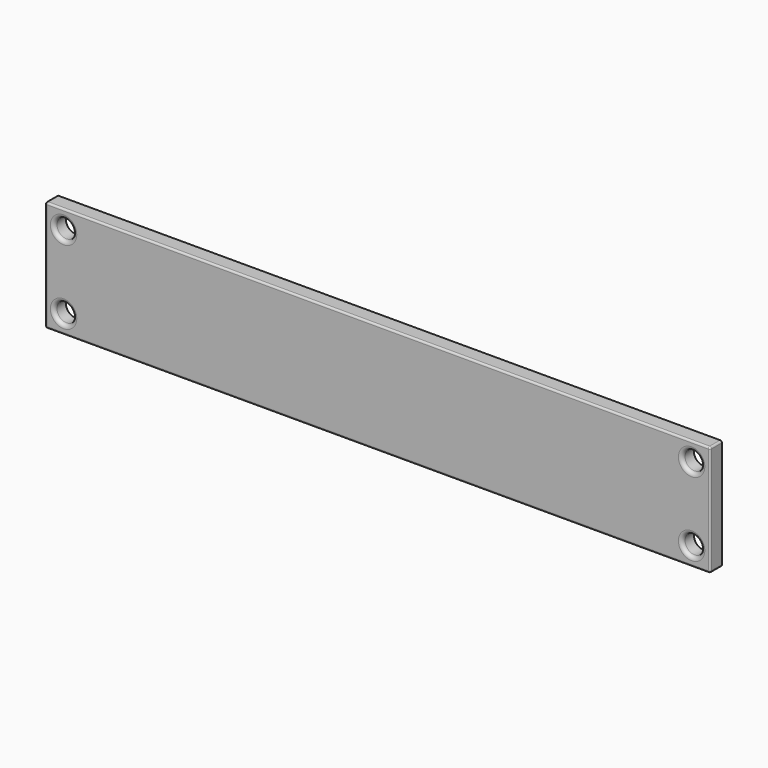
from build123d import *

# Parameters (mm, degrees)
F0_W         = 180
F0_H         = 30
F0_R         = 2.5751263091
F1_DEPTH     = 4
F2_R         = 1
F3_R         = 0.5
F4_TEXT_SIZE = 7.5757575758
F5_DEPTH     = 1


# Not quite as in the source:
# - a feature names something its author has since deleted; it is built from what else it names
# - Text() gives the source's letters only with a copy of the font that has no kerning and outlines rounded to 1/6400 em; it was checked with that copy


with BuildPart() as f1:
    # F0 (on Front) → F1 (new body)
    with BuildSketch(Plane.XZ):
        Rectangle(F0_W, F0_H)
        with Locations((-85, -10)):
            Circle(F0_R, mode=Mode.SUBTRACT)
        with Locations((85, -10)):
            Circle(F0_R, mode=Mode.SUBTRACT)
        with Locations((-85, 10)):
            Circle(F0_R, mode=Mode.SUBTRACT)
        with Locations((85, 10)):
            Circle(F0_R, mode=Mode.SUBTRACT)
    extrude(amount=F1_DEPTH)

    # F2
    f2_edges = [f1.edges().sort_by_distance(p)[0] for p in [
        (-87.575126, -4, 10),
        (-87.575126, -4, -10),
        (82.424874, -4, 10),
        (82.424874, -4, -10),
    ]]
    fillet(f2_edges, radius=F2_R)

    # F3
    f3_edges = [f1.edges().sort_by_distance(p)[0] for p in [
        (0, -4, 15),
        (-90, -4, 0),
        (0, -4, -15),
        (90, -4, 0),
        (-90, -2, 15),
        (-90, -2, -15),
        (90, -2, 15),
        (90, -2, -15),
    ]]
    fillet(f3_edges, radius=F3_R)

    # F4 (on face) → F5 (join)
    with BuildSketch(Plane(origin=(0, 0, 0), x_dir=(-1, 0, 0), z_dir=(0, 1, 0))):
        with Locations((-69.911214523, -1.4865143089)):
            Text('Berea FPSC Body', F4_TEXT_SIZE, font='Open Sans', text_align=(TextAlign.LEFT, TextAlign.BOTTOM))
    extrude(amount=F5_DEPTH)

    # F6: F1 across plane


with BuildPart() as f1_1:
    add(f1.part)
    add(f1.part.mirror(Plane.YZ))


solid = f1_1.part
